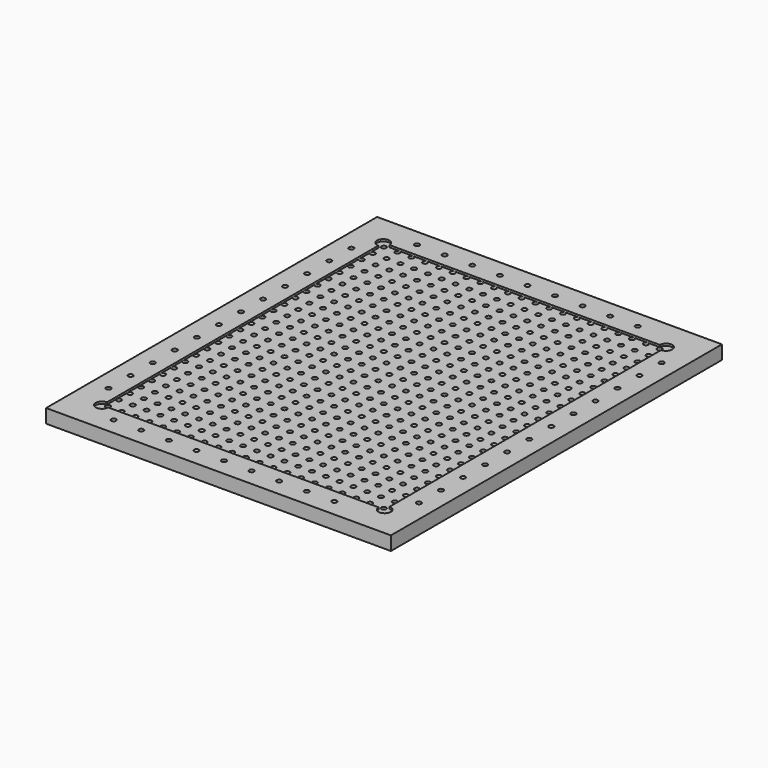
from build123d import *

# Parameters (mm, degrees)
F0_W     = 250
F0_H     = 300
F1_DEPTH = 10
F3_R     = 1.75
F4_DEPTH = 5
F5_R     = 1.75
F6_DEPTH = 5
F7_DEPTH = 1.5


with BuildPart() as f1:
    # F0 (on Top) → F1 (new body)
    with BuildSketch(Plane.XY):
        with Locations((125, 150)):
            Rectangle(F0_W, F0_H)
    extrude(amount=F1_DEPTH)

    # F3 (on face) → F4 (cut)
    with BuildSketch(Plane.XY.offset(10)):
        with Locations((24.25, 275.75)):
            Circle(F3_R)
        with Locations((24.25, 265.75)):
            Circle(F3_R)
        with Locations((24.25, 255.75)):
            Circle(F3_R)
        with Locations((24.25, 245.75)):
            Circle(F3_R)
        with Locations((24.25, 235.75)):
            Circle(F3_R)
        with Locations((24.25, 225.75)):
            Circle(F3_R)
        with Locations((24.25, 215.75)):
            Circle(F3_R)
        with Locations((24.25, 205.75)):
            Circle(F3_R)
        with Locations((24.25, 195.75)):
            Circle(F3_R)
        with Locations((24.25, 185.75)):
            Circle(F3_R)
        with Locations((24.25, 175.75)):
            Circle(F3_R)
        with Locations((24.25, 165.75)):
            Circle(F3_R)
        with Locations((24.25, 155.75)):
            Circle(F3_R)
        with Locations((24.25, 145.75)):
            Circle(F3_R)
        with Locations((24.25, 135.75)):
            Circle(F3_R)
        with Locations((24.25, 125.75)):
            Circle(F3_R)
        with Locations((24.25, 115.75)):
            Circle(F3_R)
        with Locations((24.25, 105.75)):
            Circle(F3_R)
        with Locations((24.25, 95.75)):
            Circle(F3_R)
        with Locations((24.25, 85.75)):
            Circle(F3_R)
        with Locations((24.25, 75.75)):
            Circle(F3_R)
        with Locations((24.25, 65.75)):
            Circle(F3_R)
        with Locations((24.25, 55.75)):
            Circle(F3_R)
        with Locations((24.25, 45.75)):
            Circle(F3_R)
        with Locations((24.25, 35.75)):
            Circle(F3_R)
        with Locations((24.25, 25.75)):
            Circle(F3_R)
        with Locations((34.25, 275.75)):
            Circle(F3_R)
        with Locations((34.25, 265.75)):
            Circle(F3_R)
        with Locations((34.25, 255.75)):
            Circle(F3_R)
        with Locations((34.25, 245.75)):
            Circle(F3_R)
        with Locations((34.25, 235.75)):
            Circle(F3_R)
        with Locations((34.25, 225.75)):
            Circle(F3_R)
        with Locations((34.25, 215.75)):
            Circle(F3_R)
        with Locations((34.25, 205.75)):
            Circle(F3_R)
        with Locations((34.25, 195.75)):
            Circle(F3_R)
        with Locations((34.25, 185.75)):
            Circle(F3_R)
        with Locations((34.25, 175.75)):
            Circle(F3_R)
        with Locations((34.25, 165.75)):
            Circle(F3_R)
        with Locations((34.25, 155.75)):
            Circle(F3_R)
        with Locations((34.25, 145.75)):
            Circle(F3_R)
        with Locations((34.25, 135.75)):
            Circle(F3_R)
        with Locations((34.25, 125.75)):
            Circle(F3_R)
        with Locations((34.25, 115.75)):
            Circle(F3_R)
        with Locations((34.25, 105.75)):
            Circle(F3_R)
        with Locations((34.25, 95.75)):
            Circle(F3_R)
        with Locations((34.25, 85.75)):
            Circle(F3_R)
        with Locations((34.25, 75.75)):
            Circle(F3_R)
        with Locations((34.25, 65.75)):
            Circle(F3_R)
        with Locations((34.25, 55.75)):
            Circle(F3_R)
        with Locations((34.25, 45.75)):
            Circle(F3_R)
        with Locations((34.25, 35.75)):
            Circle(F3_R)
        with Locations((34.25, 25.75)):
            Circle(F3_R)
        with Locations((44.25, 275.75)):
            Circle(F3_R)
        with Locations((44.25, 265.75)):
            Circle(F3_R)
        with Locations((44.25, 255.75)):
            Circle(F3_R)
        with Locations((44.25, 245.75)):
            Circle(F3_R)
        with Locations((44.25, 235.75)):
            Circle(F3_R)
        with Locations((44.25, 225.75)):
            Circle(F3_R)
        with Locations((44.25, 215.75)):
            Circle(F3_R)
        with Locations((44.25, 205.75)):
            Circle(F3_R)
        with Locations((44.25, 195.75)):
            Circle(F3_R)
        with Locations((44.25, 185.75)):
            Circle(F3_R)
        with Locations((44.25, 175.75)):
            Circle(F3_R)
        with Locations((44.25, 165.75)):
            Circle(F3_R)
        with Locations((44.25, 155.75)):
            Circle(F3_R)
        with Locations((44.25, 145.75)):
            Circle(F3_R)
        with Locations((44.25, 135.75)):
            Circle(F3_R)
        with Locations((44.25, 125.75)):
            Circle(F3_R)
        with Locations((44.25, 115.75)):
            Circle(F3_R)
        with Locations((44.25, 105.75)):
            Circle(F3_R)
        with Locations((44.25, 95.75)):
            Circle(F3_R)
        with Locations((44.25, 85.75)):
            Circle(F3_R)
        with Locations((44.25, 75.75)):
            Circle(F3_R)
        with Locations((44.25, 65.75)):
            Circle(F3_R)
        with Locations((44.25, 55.75)):
            Circle(F3_R)
        with Locations((44.25, 45.75)):
            Circle(F3_R)
        with Locations((44.25, 35.75)):
            Circle(F3_R)
        with Locations((44.25, 25.75)):
            Circle(F3_R)
        with Locations((54.25, 275.75)):
            Circle(F3_R)
        with Locations((54.25, 265.75)):
            Circle(F3_R)
        with Locations((54.25, 255.75)):
            Circle(F3_R)
        with Locations((54.25, 245.75)):
            Circle(F3_R)
        with Locations((54.25, 235.75)):
            Circle(F3_R)
        with Locations((54.25, 225.75)):
            Circle(F3_R)
        with Locations((54.25, 215.75)):
            Circle(F3_R)
        with Locations((54.25, 205.75)):
            Circle(F3_R)
        with Locations((54.25, 195.75)):
            Circle(F3_R)
        with Locations((54.25, 185.75)):
            Circle(F3_R)
        with Locations((54.25, 175.75)):
            Circle(F3_R)
        with Locations((54.25, 165.75)):
            Circle(F3_R)
        with Locations((54.25, 155.75)):
            Circle(F3_R)
        with Locations((54.25, 145.75)):
            Circle(F3_R)
        with Locations((54.25, 135.75)):
            Circle(F3_R)
        with Locations((54.25, 125.75)):
            Circle(F3_R)
        with Locations((54.25, 115.75)):
            Circle(F3_R)
        with Locations((54.25, 105.75)):
            Circle(F3_R)
        with Locations((54.25, 95.75)):
            Circle(F3_R)
        with Locations((54.25, 85.75)):
            Circle(F3_R)
        with Locations((54.25, 75.75)):
            Circle(F3_R)
        with Locations((54.25, 65.75)):
            Circle(F3_R)
        with Locations((54.25, 55.75)):
            Circle(F3_R)
        with Locations((54.25, 45.75)):
            Circle(F3_R)
        with Locations((54.25, 35.75)):
            Circle(F3_R)
        with Locations((54.25, 25.75)):
            Circle(F3_R)
        with Locations((64.25, 275.75)):
            Circle(F3_R)
        with Locations((64.25, 265.75)):
            Circle(F3_R)
        with Locations((64.25, 255.75)):
            Circle(F3_R)
        with Locations((64.25, 245.75)):
            Circle(F3_R)
        with Locations((64.25, 235.75)):
            Circle(F3_R)
        with Locations((64.25, 225.75)):
            Circle(F3_R)
        with Locations((64.25, 215.75)):
            Circle(F3_R)
        with Locations((64.25, 205.75)):
            Circle(F3_R)
        with Locations((64.25, 195.75)):
            Circle(F3_R)
        with Locations((64.25, 185.75)):
            Circle(F3_R)
        with Locations((64.25, 175.75)):
            Circle(F3_R)
        with Locations((64.25, 165.75)):
            Circle(F3_R)
        with Locations((64.25, 155.75)):
            Circle(F3_R)
        with Locations((64.25, 145.75)):
            Circle(F3_R)
        with Locations((64.25, 135.75)):
            Circle(F3_R)
        with Locations((64.25, 125.75)):
            Circle(F3_R)
        with Locations((64.25, 115.75)):
            Circle(F3_R)
        with Locations((64.25, 105.75)):
            Circle(F3_R)
        with Locations((64.25, 95.75)):
            Circle(F3_R)
        with Locations((64.25, 85.75)):
            Circle(F3_R)
        with Locations((64.25, 75.75)):
            Circle(F3_R)
        with Locations((64.25, 65.75)):
            Circle(F3_R)
        with Locations((64.25, 55.75)):
            Circle(F3_R)
        with Locations((64.25, 45.75)):
            Circle(F3_R)
        with Locations((64.25, 35.75)):
            Circle(F3_R)
        with Locations((64.25, 25.75)):
            Circle(F3_R)
        with Locations((74.25, 275.75)):
            Circle(F3_R)
        with Locations((74.25, 265.75)):
            Circle(F3_R)
        with Locations((74.25, 255.75)):
            Circle(F3_R)
        with Locations((74.25, 245.75)):
            Circle(F3_R)
        with Locations((74.25, 235.75)):
            Circle(F3_R)
        with Locations((74.25, 225.75)):
            Circle(F3_R)
        with Locations((74.25, 215.75)):
            Circle(F3_R)
        with Locations((74.25, 205.75)):
            Circle(F3_R)
        with Locations((74.25, 195.75)):
            Circle(F3_R)
        with Locations((74.25, 185.75)):
            Circle(F3_R)
        with Locations((74.25, 175.75)):
            Circle(F3_R)
        with Locations((74.25, 165.75)):
            Circle(F3_R)
        with Locations((74.25, 155.75)):
            Circle(F3_R)
        with Locations((74.25, 145.75)):
            Circle(F3_R)
        with Locations((74.25, 135.75)):
            Circle(F3_R)
        with Locations((74.25, 125.75)):
            Circle(F3_R)
        with Locations((74.25, 115.75)):
            Circle(F3_R)
        with Locations((74.25, 105.75)):
            Circle(F3_R)
        with Locations((74.25, 95.75)):
            Circle(F3_R)
        with Locations((74.25, 85.75)):
            Circle(F3_R)
        with Locations((74.25, 75.75)):
            Circle(F3_R)
        with Locations((74.25, 65.75)):
            Circle(F3_R)
        with Locations((74.25, 55.75)):
            Circle(F3_R)
        with Locations((74.25, 45.75)):
            Circle(F3_R)
        with Locations((74.25, 35.75)):
            Circle(F3_R)
        with Locations((74.25, 25.75)):
            Circle(F3_R)
        with Locations((84.25, 275.75)):
            Circle(F3_R)
        with Locations((84.25, 265.75)):
            Circle(F3_R)
        with Locations((84.25, 255.75)):
            Circle(F3_R)
        with Locations((84.25, 245.75)):
            Circle(F3_R)
        with Locations((84.25, 235.75)):
            Circle(F3_R)
        with Locations((84.25, 225.75)):
            Circle(F3_R)
        with Locations((84.25, 215.75)):
            Circle(F3_R)
        with Locations((84.25, 205.75)):
            Circle(F3_R)
        with Locations((84.25, 195.75)):
            Circle(F3_R)
        with Locations((84.25, 185.75)):
            Circle(F3_R)
        with Locations((84.25, 175.75)):
            Circle(F3_R)
        with Locations((84.25, 165.75)):
            Circle(F3_R)
        with Locations((84.25, 155.75)):
            Circle(F3_R)
        with Locations((84.25, 145.75)):
            Circle(F3_R)
        with Locations((84.25, 135.75)):
            Circle(F3_R)
        with Locations((84.25, 125.75)):
            Circle(F3_R)
        with Locations((84.25, 115.75)):
            Circle(F3_R)
        with Locations((84.25, 105.75)):
            Circle(F3_R)
        with Locations((84.25, 95.75)):
            Circle(F3_R)
        with Locations((84.25, 85.75)):
            Circle(F3_R)
        with Locations((84.25, 75.75)):
            Circle(F3_R)
        with Locations((84.25, 65.75)):
            Circle(F3_R)
        with Locations((84.25, 55.75)):
            Circle(F3_R)
        with Locations((84.25, 45.75)):
            Circle(F3_R)
        with Locations((84.25, 35.75)):
            Circle(F3_R)
        with Locations((84.25, 25.75)):
            Circle(F3_R)
        with Locations((94.25, 275.75)):
            Circle(F3_R)
        with Locations((94.25, 265.75)):
            Circle(F3_R)
        with Locations((94.25, 255.75)):
            Circle(F3_R)
        with Locations((94.25, 245.75)):
            Circle(F3_R)
        with Locations((94.25, 235.75)):
            Circle(F3_R)
        with Locations((94.25, 225.75)):
            Circle(F3_R)
        with Locations((94.25, 215.75)):
            Circle(F3_R)
        with Locations((94.25, 205.75)):
            Circle(F3_R)
        with Locations((94.25, 195.75)):
            Circle(F3_R)
        with Locations((94.25, 185.75)):
            Circle(F3_R)
        with Locations((94.25, 175.75)):
            Circle(F3_R)
        with Locations((94.25, 165.75)):
            Circle(F3_R)
        with Locations((94.25, 155.75)):
            Circle(F3_R)
        with Locations((94.25, 145.75)):
            Circle(F3_R)
        with Locations((94.25, 135.75)):
            Circle(F3_R)
        with Locations((94.25, 125.75)):
            Circle(F3_R)
        with Locations((94.25, 115.75)):
            Circle(F3_R)
        with Locations((94.25, 105.75)):
            Circle(F3_R)
        with Locations((94.25, 95.75)):
            Circle(F3_R)
        with Locations((94.25, 85.75)):
            Circle(F3_R)
        with Locations((94.25, 75.75)):
            Circle(F3_R)
        with Locations((94.25, 65.75)):
            Circle(F3_R)
        with Locations((94.25, 55.75)):
            Circle(F3_R)
        with Locations((94.25, 45.75)):
            Circle(F3_R)
        with Locations((94.25, 35.75)):
            Circle(F3_R)
        with Locations((94.25, 25.75)):
            Circle(F3_R)
        with Locations((104.25, 275.75)):
            Circle(F3_R)
        with Locations((104.25, 265.75)):
            Circle(F3_R)
        with Locations((104.25, 255.75)):
            Circle(F3_R)
        with Locations((104.25, 245.75)):
            Circle(F3_R)
        with Locations((104.25, 235.75)):
            Circle(F3_R)
        with Locations((104.25, 225.75)):
            Circle(F3_R)
        with Locations((104.25, 215.75)):
            Circle(F3_R)
        with Locations((104.25, 205.75)):
            Circle(F3_R)
        with Locations((104.25, 195.75)):
            Circle(F3_R)
        with Locations((104.25, 185.75)):
            Circle(F3_R)
        with Locations((104.25, 175.75)):
            Circle(F3_R)
        with Locations((104.25, 165.75)):
            Circle(F3_R)
        with Locations((104.25, 155.75)):
            Circle(F3_R)
        with Locations((104.25, 145.75)):
            Circle(F3_R)
        with Locations((104.25, 135.75)):
            Circle(F3_R)
        with Locations((104.25, 125.75)):
            Circle(F3_R)
        with Locations((104.25, 115.75)):
            Circle(F3_R)
        with Locations((104.25, 105.75)):
            Circle(F3_R)
        with Locations((104.25, 95.75)):
            Circle(F3_R)
        with Locations((104.25, 85.75)):
            Circle(F3_R)
        with Locations((104.25, 75.75)):
            Circle(F3_R)
        with Locations((104.25, 65.75)):
            Circle(F3_R)
        with Locations((104.25, 55.75)):
            Circle(F3_R)
        with Locations((104.25, 45.75)):
            Circle(F3_R)
        with Locations((104.25, 35.75)):
            Circle(F3_R)
        with Locations((104.25, 25.75)):
            Circle(F3_R)
        with Locations((114.25, 275.75)):
            Circle(F3_R)
        with Locations((114.25, 265.75)):
            Circle(F3_R)
        with Locations((114.25, 255.75)):
            Circle(F3_R)
        with Locations((114.25, 245.75)):
            Circle(F3_R)
        with Locations((114.25, 235.75)):
            Circle(F3_R)
        with Locations((114.25, 225.75)):
            Circle(F3_R)
        with Locations((114.25, 215.75)):
            Circle(F3_R)
        with Locations((114.25, 205.75)):
            Circle(F3_R)
        with Locations((114.25, 195.75)):
            Circle(F3_R)
        with Locations((114.25, 185.75)):
            Circle(F3_R)
        with Locations((114.25, 175.75)):
            Circle(F3_R)
        with Locations((114.25, 165.75)):
            Circle(F3_R)
        with Locations((114.25, 155.75)):
            Circle(F3_R)
        with Locations((114.25, 145.75)):
            Circle(F3_R)
        with Locations((114.25, 135.75)):
            Circle(F3_R)
        with Locations((114.25, 125.75)):
            Circle(F3_R)
        with Locations((114.25, 115.75)):
            Circle(F3_R)
        with Locations((114.25, 105.75)):
            Circle(F3_R)
        with Locations((114.25, 95.75)):
            Circle(F3_R)
        with Locations((114.25, 85.75)):
            Circle(F3_R)
        with Locations((114.25, 75.75)):
            Circle(F3_R)
        with Locations((114.25, 65.75)):
            Circle(F3_R)
        with Locations((114.25, 55.75)):
            Circle(F3_R)
        with Locations((114.25, 45.75)):
            Circle(F3_R)
        with Locations((114.25, 35.75)):
            Circle(F3_R)
        with Locations((114.25, 25.75)):
            Circle(F3_R)
        with Locations((124.25, 275.75)):
            Circle(F3_R)
        with Locations((124.25, 265.75)):
            Circle(F3_R)
        with Locations((124.25, 255.75)):
            Circle(F3_R)
        with Locations((124.25, 245.75)):
            Circle(F3_R)
        with Locations((124.25, 235.75)):
            Circle(F3_R)
        with Locations((124.25, 225.75)):
            Circle(F3_R)
        with Locations((124.25, 215.75)):
            Circle(F3_R)
        with Locations((124.25, 205.75)):
            Circle(F3_R)
        with Locations((124.25, 195.75)):
            Circle(F3_R)
        with Locations((124.25, 185.75)):
            Circle(F3_R)
        with Locations((124.25, 175.75)):
            Circle(F3_R)
        with Locations((124.25, 165.75)):
            Circle(F3_R)
        with Locations((124.25, 155.75)):
            Circle(F3_R)
        with Locations((124.25, 145.75)):
            Circle(F3_R)
        with Locations((124.25, 135.75)):
            Circle(F3_R)
        with Locations((124.25, 125.75)):
            Circle(F3_R)
        with Locations((124.25, 115.75)):
            Circle(F3_R)
        with Locations((124.25, 105.75)):
            Circle(F3_R)
        with Locations((124.25, 95.75)):
            Circle(F3_R)
        with Locations((124.25, 85.75)):
            Circle(F3_R)
        with Locations((124.25, 75.75)):
            Circle(F3_R)
        with Locations((124.25, 65.75)):
            Circle(F3_R)
        with Locations((124.25, 55.75)):
            Circle(F3_R)
        with Locations((124.25, 45.75)):
            Circle(F3_R)
        with Locations((124.25, 35.75)):
            Circle(F3_R)
        with Locations((124.25, 25.75)):
            Circle(F3_R)
        with Locations((134.25, 275.75)):
            Circle(F3_R)
        with Locations((134.25, 265.75)):
            Circle(F3_R)
        with Locations((134.25, 255.75)):
            Circle(F3_R)
        with Locations((134.25, 245.75)):
            Circle(F3_R)
        with Locations((134.25, 235.75)):
            Circle(F3_R)
        with Locations((134.25, 225.75)):
            Circle(F3_R)
        with Locations((134.25, 215.75)):
            Circle(F3_R)
        with Locations((134.25, 205.75)):
            Circle(F3_R)
        with Locations((134.25, 195.75)):
            Circle(F3_R)
        with Locations((134.25, 185.75)):
            Circle(F3_R)
        with Locations((134.25, 175.75)):
            Circle(F3_R)
        with Locations((134.25, 165.75)):
            Circle(F3_R)
        with Locations((134.25, 155.75)):
            Circle(F3_R)
        with Locations((134.25, 145.75)):
            Circle(F3_R)
        with Locations((134.25, 135.75)):
            Circle(F3_R)
        with Locations((134.25, 125.75)):
            Circle(F3_R)
        with Locations((134.25, 115.75)):
            Circle(F3_R)
        with Locations((134.25, 105.75)):
            Circle(F3_R)
        with Locations((134.25, 95.75)):
            Circle(F3_R)
        with Locations((134.25, 85.75)):
            Circle(F3_R)
        with Locations((134.25, 75.75)):
            Circle(F3_R)
        with Locations((134.25, 65.75)):
            Circle(F3_R)
        with Locations((134.25, 55.75)):
            Circle(F3_R)
        with Locations((134.25, 45.75)):
            Circle(F3_R)
        with Locations((134.25, 35.75)):
            Circle(F3_R)
        with Locations((134.25, 25.75)):
            Circle(F3_R)
        with Locations((144.25, 275.75)):
            Circle(F3_R)
        with Locations((144.25, 265.75)):
            Circle(F3_R)
        with Locations((144.25, 255.75)):
            Circle(F3_R)
        with Locations((144.25, 245.75)):
            Circle(F3_R)
        with Locations((144.25, 235.75)):
            Circle(F3_R)
        with Locations((144.25, 225.75)):
            Circle(F3_R)
        with Locations((144.25, 215.75)):
            Circle(F3_R)
        with Locations((144.25, 205.75)):
            Circle(F3_R)
        with Locations((144.25, 195.75)):
            Circle(F3_R)
        with Locations((144.25, 185.75)):
            Circle(F3_R)
        with Locations((144.25, 175.75)):
            Circle(F3_R)
        with Locations((144.25, 165.75)):
            Circle(F3_R)
        with Locations((144.25, 155.75)):
            Circle(F3_R)
        with Locations((144.25, 145.75)):
            Circle(F3_R)
        with Locations((144.25, 135.75)):
            Circle(F3_R)
        with Locations((144.25, 125.75)):
            Circle(F3_R)
        with Locations((144.25, 115.75)):
            Circle(F3_R)
        with Locations((144.25, 105.75)):
            Circle(F3_R)
        with Locations((144.25, 95.75)):
            Circle(F3_R)
        with Locations((144.25, 85.75)):
            Circle(F3_R)
        with Locations((144.25, 75.75)):
            Circle(F3_R)
        with Locations((144.25, 65.75)):
            Circle(F3_R)
        with Locations((144.25, 55.75)):
            Circle(F3_R)
        with Locations((144.25, 45.75)):
            Circle(F3_R)
        with Locations((144.25, 35.75)):
            Circle(F3_R)
        with Locations((144.25, 25.75)):
            Circle(F3_R)
        with Locations((154.25, 275.75)):
            Circle(F3_R)
        with Locations((154.25, 265.75)):
            Circle(F3_R)
        with Locations((154.25, 255.75)):
            Circle(F3_R)
        with Locations((154.25, 245.75)):
            Circle(F3_R)
        with Locations((154.25, 235.75)):
            Circle(F3_R)
        with Locations((154.25, 225.75)):
            Circle(F3_R)
        with Locations((154.25, 215.75)):
            Circle(F3_R)
        with Locations((154.25, 205.75)):
            Circle(F3_R)
        with Locations((154.25, 195.75)):
            Circle(F3_R)
        with Locations((154.25, 185.75)):
            Circle(F3_R)
        with Locations((154.25, 175.75)):
            Circle(F3_R)
        with Locations((154.25, 165.75)):
            Circle(F3_R)
        with Locations((154.25, 155.75)):
            Circle(F3_R)
        with Locations((154.25, 145.75)):
            Circle(F3_R)
        with Locations((154.25, 135.75)):
            Circle(F3_R)
        with Locations((154.25, 125.75)):
            Circle(F3_R)
        with Locations((154.25, 115.75)):
            Circle(F3_R)
        with Locations((154.25, 105.75)):
            Circle(F3_R)
        with Locations((154.25, 95.75)):
            Circle(F3_R)
        with Locations((154.25, 85.75)):
            Circle(F3_R)
        with Locations((154.25, 75.75)):
            Circle(F3_R)
        with Locations((154.25, 65.75)):
            Circle(F3_R)
        with Locations((154.25, 55.75)):
            Circle(F3_R)
        with Locations((154.25, 45.75)):
            Circle(F3_R)
        with Locations((154.25, 35.75)):
            Circle(F3_R)
        with Locations((154.25, 25.75)):
            Circle(F3_R)
        with Locations((164.25, 275.75)):
            Circle(F3_R)
        with Locations((164.25, 265.75)):
            Circle(F3_R)
        with Locations((164.25, 255.75)):
            Circle(F3_R)
        with Locations((164.25, 245.75)):
            Circle(F3_R)
        with Locations((164.25, 235.75)):
            Circle(F3_R)
        with Locations((164.25, 225.75)):
            Circle(F3_R)
        with Locations((164.25, 215.75)):
            Circle(F3_R)
        with Locations((164.25, 205.75)):
            Circle(F3_R)
        with Locations((164.25, 195.75)):
            Circle(F3_R)
        with Locations((164.25, 185.75)):
            Circle(F3_R)
        with Locations((164.25, 175.75)):
            Circle(F3_R)
        with Locations((164.25, 165.75)):
            Circle(F3_R)
        with Locations((164.25, 155.75)):
            Circle(F3_R)
        with Locations((164.25, 145.75)):
            Circle(F3_R)
        with Locations((164.25, 135.75)):
            Circle(F3_R)
        with Locations((164.25, 125.75)):
            Circle(F3_R)
        with Locations((164.25, 115.75)):
            Circle(F3_R)
        with Locations((164.25, 105.75)):
            Circle(F3_R)
        with Locations((164.25, 95.75)):
            Circle(F3_R)
        with Locations((164.25, 85.75)):
            Circle(F3_R)
        with Locations((164.25, 75.75)):
            Circle(F3_R)
        with Locations((164.25, 65.75)):
            Circle(F3_R)
        with Locations((164.25, 55.75)):
            Circle(F3_R)
        with Locations((164.25, 45.75)):
            Circle(F3_R)
        with Locations((164.25, 35.75)):
            Circle(F3_R)
        with Locations((164.25, 25.75)):
            Circle(F3_R)
        with Locations((174.25, 275.75)):
            Circle(F3_R)
        with Locations((174.25, 265.75)):
            Circle(F3_R)
        with Locations((174.25, 255.75)):
            Circle(F3_R)
        with Locations((174.25, 245.75)):
            Circle(F3_R)
        with Locations((174.25, 235.75)):
            Circle(F3_R)
        with Locations((174.25, 225.75)):
            Circle(F3_R)
        with Locations((174.25, 215.75)):
            Circle(F3_R)
        with Locations((174.25, 205.75)):
            Circle(F3_R)
        with Locations((174.25, 195.75)):
            Circle(F3_R)
        with Locations((174.25, 185.75)):
            Circle(F3_R)
        with Locations((174.25, 175.75)):
            Circle(F3_R)
        with Locations((174.25, 165.75)):
            Circle(F3_R)
        with Locations((174.25, 155.75)):
            Circle(F3_R)
        with Locations((174.25, 145.75)):
            Circle(F3_R)
        with Locations((174.25, 135.75)):
            Circle(F3_R)
        with Locations((174.25, 125.75)):
            Circle(F3_R)
        with Locations((174.25, 115.75)):
            Circle(F3_R)
        with Locations((174.25, 105.75)):
            Circle(F3_R)
        with Locations((174.25, 95.75)):
            Circle(F3_R)
        with Locations((174.25, 85.75)):
            Circle(F3_R)
        with Locations((174.25, 75.75)):
            Circle(F3_R)
        with Locations((174.25, 65.75)):
            Circle(F3_R)
        with Locations((174.25, 55.75)):
            Circle(F3_R)
        with Locations((174.25, 45.75)):
            Circle(F3_R)
        with Locations((174.25, 35.75)):
            Circle(F3_R)
        with Locations((174.25, 25.75)):
            Circle(F3_R)
        with Locations((184.25, 275.75)):
            Circle(F3_R)
        with Locations((184.25, 265.75)):
            Circle(F3_R)
        with Locations((184.25, 255.75)):
            Circle(F3_R)
        with Locations((184.25, 245.75)):
            Circle(F3_R)
        with Locations((184.25, 235.75)):
            Circle(F3_R)
        with Locations((184.25, 225.75)):
            Circle(F3_R)
        with Locations((184.25, 215.75)):
            Circle(F3_R)
        with Locations((184.25, 205.75)):
            Circle(F3_R)
        with Locations((184.25, 195.75)):
            Circle(F3_R)
        with Locations((184.25, 185.75)):
            Circle(F3_R)
        with Locations((184.25, 175.75)):
            Circle(F3_R)
        with Locations((184.25, 165.75)):
            Circle(F3_R)
        with Locations((184.25, 155.75)):
            Circle(F3_R)
        with Locations((184.25, 145.75)):
            Circle(F3_R)
        with Locations((184.25, 135.75)):
            Circle(F3_R)
        with Locations((184.25, 125.75)):
            Circle(F3_R)
        with Locations((184.25, 115.75)):
            Circle(F3_R)
        with Locations((184.25, 105.75)):
            Circle(F3_R)
        with Locations((184.25, 95.75)):
            Circle(F3_R)
        with Locations((184.25, 85.75)):
            Circle(F3_R)
        with Locations((184.25, 75.75)):
            Circle(F3_R)
        with Locations((184.25, 65.75)):
            Circle(F3_R)
        with Locations((184.25, 55.75)):
            Circle(F3_R)
        with Locations((184.25, 45.75)):
            Circle(F3_R)
        with Locations((184.25, 35.75)):
            Circle(F3_R)
        with Locations((184.25, 25.75)):
            Circle(F3_R)
        with Locations((194.25, 275.75)):
            Circle(F3_R)
        with Locations((194.25, 265.75)):
            Circle(F3_R)
        with Locations((194.25, 255.75)):
            Circle(F3_R)
        with Locations((194.25, 245.75)):
            Circle(F3_R)
        with Locations((194.25, 235.75)):
            Circle(F3_R)
        with Locations((194.25, 225.75)):
            Circle(F3_R)
        with Locations((194.25, 215.75)):
            Circle(F3_R)
        with Locations((194.25, 205.75)):
            Circle(F3_R)
        with Locations((194.25, 195.75)):
            Circle(F3_R)
        with Locations((194.25, 185.75)):
            Circle(F3_R)
        with Locations((194.25, 175.75)):
            Circle(F3_R)
        with Locations((194.25, 165.75)):
            Circle(F3_R)
        with Locations((194.25, 155.75)):
            Circle(F3_R)
        with Locations((194.25, 145.75)):
            Circle(F3_R)
        with Locations((194.25, 135.75)):
            Circle(F3_R)
        with Locations((194.25, 125.75)):
            Circle(F3_R)
        with Locations((194.25, 115.75)):
            Circle(F3_R)
        with Locations((194.25, 105.75)):
            Circle(F3_R)
        with Locations((194.25, 95.75)):
            Circle(F3_R)
        with Locations((194.25, 85.75)):
            Circle(F3_R)
        with Locations((194.25, 75.75)):
            Circle(F3_R)
        with Locations((194.25, 65.75)):
            Circle(F3_R)
        with Locations((194.25, 55.75)):
            Circle(F3_R)
        with Locations((194.25, 45.75)):
            Circle(F3_R)
        with Locations((194.25, 35.75)):
            Circle(F3_R)
        with Locations((194.25, 25.75)):
            Circle(F3_R)
        with Locations((204.25, 275.75)):
            Circle(F3_R)
        with Locations((204.25, 265.75)):
            Circle(F3_R)
        with Locations((204.25, 255.75)):
            Circle(F3_R)
        with Locations((204.25, 245.75)):
            Circle(F3_R)
        with Locations((204.25, 235.75)):
            Circle(F3_R)
        with Locations((204.25, 225.75)):
            Circle(F3_R)
        with Locations((204.25, 215.75)):
            Circle(F3_R)
        with Locations((204.25, 205.75)):
            Circle(F3_R)
        with Locations((204.25, 195.75)):
            Circle(F3_R)
        with Locations((204.25, 185.75)):
            Circle(F3_R)
        with Locations((204.25, 175.75)):
            Circle(F3_R)
        with Locations((204.25, 165.75)):
            Circle(F3_R)
        with Locations((204.25, 155.75)):
            Circle(F3_R)
        with Locations((204.25, 145.75)):
            Circle(F3_R)
        with Locations((204.25, 135.75)):
            Circle(F3_R)
        with Locations((204.25, 125.75)):
            Circle(F3_R)
        with Locations((204.25, 115.75)):
            Circle(F3_R)
        with Locations((204.25, 105.75)):
            Circle(F3_R)
        with Locations((204.25, 95.75)):
            Circle(F3_R)
        with Locations((204.25, 85.75)):
            Circle(F3_R)
        with Locations((204.25, 75.75)):
            Circle(F3_R)
        with Locations((204.25, 65.75)):
            Circle(F3_R)
        with Locations((204.25, 55.75)):
            Circle(F3_R)
        with Locations((204.25, 45.75)):
            Circle(F3_R)
        with Locations((204.25, 35.75)):
            Circle(F3_R)
        with Locations((204.25, 25.75)):
            Circle(F3_R)
        with Locations((214.25, 275.75)):
            Circle(F3_R)
        with Locations((214.25, 265.75)):
            Circle(F3_R)
        with Locations((214.25, 255.75)):
            Circle(F3_R)
        with Locations((214.25, 245.75)):
            Circle(F3_R)
        with Locations((214.25, 235.75)):
            Circle(F3_R)
        with Locations((214.25, 225.75)):
            Circle(F3_R)
        with Locations((214.25, 215.75)):
            Circle(F3_R)
        with Locations((214.25, 205.75)):
            Circle(F3_R)
        with Locations((214.25, 195.75)):
            Circle(F3_R)
        with Locations((214.25, 185.75)):
            Circle(F3_R)
        with Locations((214.25, 175.75)):
            Circle(F3_R)
        with Locations((214.25, 165.75)):
            Circle(F3_R)
        with Locations((214.25, 155.75)):
            Circle(F3_R)
        with Locations((214.25, 145.75)):
            Circle(F3_R)
        with Locations((214.25, 135.75)):
            Circle(F3_R)
        with Locations((214.25, 125.75)):
            Circle(F3_R)
        with Locations((214.25, 115.75)):
            Circle(F3_R)
        with Locations((214.25, 105.75)):
            Circle(F3_R)
        with Locations((214.25, 95.75)):
            Circle(F3_R)
        with Locations((214.25, 85.75)):
            Circle(F3_R)
        with Locations((214.25, 75.75)):
            Circle(F3_R)
        with Locations((214.25, 65.75)):
            Circle(F3_R)
        with Locations((214.25, 55.75)):
            Circle(F3_R)
        with Locations((214.25, 45.75)):
            Circle(F3_R)
        with Locations((214.25, 35.75)):
            Circle(F3_R)
        with Locations((214.25, 25.75)):
            Circle(F3_R)
        with Locations((224.25, 275.75)):
            Circle(F3_R)
        with Locations((224.25, 265.75)):
            Circle(F3_R)
        with Locations((224.25, 255.75)):
            Circle(F3_R)
        with Locations((224.25, 245.75)):
            Circle(F3_R)
        with Locations((224.25, 235.75)):
            Circle(F3_R)
        with Locations((224.25, 225.75)):
            Circle(F3_R)
        with Locations((224.25, 215.75)):
            Circle(F3_R)
        with Locations((224.25, 205.75)):
            Circle(F3_R)
        with Locations((224.25, 195.75)):
            Circle(F3_R)
        with Locations((224.25, 185.75)):
            Circle(F3_R)
        with Locations((224.25, 175.75)):
            Circle(F3_R)
        with Locations((224.25, 165.75)):
            Circle(F3_R)
        with Locations((224.25, 155.75)):
            Circle(F3_R)
        with Locations((224.25, 145.75)):
            Circle(F3_R)
        with Locations((224.25, 135.75)):
            Circle(F3_R)
        with Locations((224.25, 125.75)):
            Circle(F3_R)
        with Locations((224.25, 115.75)):
            Circle(F3_R)
        with Locations((224.25, 105.75)):
            Circle(F3_R)
        with Locations((224.25, 95.75)):
            Circle(F3_R)
        with Locations((224.25, 85.75)):
            Circle(F3_R)
        with Locations((224.25, 75.75)):
            Circle(F3_R)
        with Locations((224.25, 65.75)):
            Circle(F3_R)
        with Locations((224.25, 55.75)):
            Circle(F3_R)
        with Locations((224.25, 45.75)):
            Circle(F3_R)
        with Locations((224.25, 35.75)):
            Circle(F3_R)
        with Locations((224.25, 25.75)):
            Circle(F3_R)
    extrude(amount=-F4_DEPTH, mode=Mode.SUBTRACT)

    # F5 (on face) → F6 (cut)
    with BuildSketch(Plane.XY.offset(10)):
        with Locations((39, 287.5)):
            Circle(F5_R)
        with Locations((39, 12.5)):
            Circle(F5_R)
        with Locations((59, 287.5)):
            Circle(F5_R)
        with Locations((59, 12.5)):
            Circle(F5_R)
        with Locations((79, 287.5)):
            Circle(F5_R)
        with Locations((79, 12.5)):
            Circle(F5_R)
        with Locations((99, 287.5)):
            Circle(F5_R)
        with Locations((99, 12.5)):
            Circle(F5_R)
        with Locations((119, 287.5)):
            Circle(F5_R)
        with Locations((119, 12.5)):
            Circle(F5_R)
        with Locations((139, 287.5)):
            Circle(F5_R)
        with Locations((139, 12.5)):
            Circle(F5_R)
        with Locations((159, 287.5)):
            Circle(F5_R)
        with Locations((159, 12.5)):
            Circle(F5_R)
        with Locations((179, 287.5)):
            Circle(F5_R)
        with Locations((179, 12.5)):
            Circle(F5_R)
        with Locations((199, 287.5)):
            Circle(F5_R)
        with Locations((199, 12.5)):
            Circle(F5_R)
        with Locations((12.5, 261)):
            Circle(F5_R)
        with Locations((12.5, 241)):
            Circle(F5_R)
        with Locations((12.5, 221)):
            Circle(F5_R)
        with Locations((12.5, 201)):
            Circle(F5_R)
        with Locations((12.5, 181)):
            Circle(F5_R)
        with Locations((12.5, 161)):
            Circle(F5_R)
        with Locations((12.5, 141)):
            Circle(F5_R)
        with Locations((12.5, 121)):
            Circle(F5_R)
        with Locations((12.5, 101)):
            Circle(F5_R)
        with Locations((12.5, 81)):
            Circle(F5_R)
        with Locations((12.5, 61)):
            Circle(F5_R)
        with Locations((12.5, 41)):
            Circle(F5_R)
        with Locations((237.5, 261)):
            Circle(F5_R)
        with Locations((237.5, 241)):
            Circle(F5_R)
        with Locations((237.5, 221)):
            Circle(F5_R)
        with Locations((237.5, 201)):
            Circle(F5_R)
        with Locations((237.5, 181)):
            Circle(F5_R)
        with Locations((237.5, 161)):
            Circle(F5_R)
        with Locations((237.5, 141)):
            Circle(F5_R)
        with Locations((237.5, 121)):
            Circle(F5_R)
        with Locations((237.5, 101)):
            Circle(F5_R)
        with Locations((237.5, 81)):
            Circle(F5_R)
        with Locations((237.5, 61)):
            Circle(F5_R)
        with Locations((237.5, 41)):
            Circle(F5_R)
    extrude(amount=-F6_DEPTH, mode=Mode.SUBTRACT)

    # F2 (on face) → F7 (cut)
    with BuildSketch(Plane.XY.offset(10)):
        with BuildLine():
            Line((22.5, 273), (22.5, 277.5))
            Line((22.5, 277.5), (27, 277.5))
            ThreePointArc((27, 277.5), (19.3180194847, 280.6819805153), (22.5, 273))
        make_face()
        with BuildLine():
            Line((27, 277.5), (22.5, 277.5))
            Line((22.5, 277.5), (22.5, 273))
            ThreePointArc((22.5, 273), (25.6819805153, 274.3180194847), (27, 277.5))
        make_face()
        with BuildLine():
            Line((223, 277.5), (27, 277.5))
            ThreePointArc((27, 277.5), (25.6819805153, 274.3180194847), (22.5, 273))
            Line((22.5, 273), (22.5, 27))
            ThreePointArc((22.5, 27), (25.6819805153, 25.6819805153), (27, 22.5))
            Line((27, 22.5), (223, 22.5))
            ThreePointArc((223, 22.5), (224.3180194847, 25.6819805153), (227.5, 27))
            Line((227.5, 27), (227.5, 273))
            ThreePointArc((227.5, 273), (224.3180194847, 274.3180194847), (223, 277.5))
        make_face()
        with BuildLine():
            ThreePointArc((232, 277.5), (227.5, 282), (223, 277.5))
            Line((223, 277.5), (227.5, 277.5))
            Line((227.5, 277.5), (227.5, 273))
            ThreePointArc((227.5, 273), (230.6819805153, 274.3180194847), (232, 277.5))
        make_face()
        with BuildLine():
            Line((227.5, 277.5), (223, 277.5))
            ThreePointArc((223, 277.5), (224.3180194847, 274.3180194847), (227.5, 273))
            Line((227.5, 273), (227.5, 277.5))
        make_face()
        with BuildLine():
            ThreePointArc((27, 22.5), (25.6819805153, 25.6819805153), (22.5, 27))
            Line((22.5, 27), (22.5, 22.5))
            Line((22.5, 22.5), (27, 22.5))
        make_face()
        with BuildLine():
            Line((22.5, 22.5), (22.5, 27))
            ThreePointArc((22.5, 27), (19.3180194847, 19.3180194847), (27, 22.5))
            Line((27, 22.5), (22.5, 22.5))
        make_face()
        with BuildLine():
            ThreePointArc((232, 22.5), (230.6819805153, 25.6819805153), (227.5, 27))
            Line((227.5, 27), (227.5, 22.5))
            Line((227.5, 22.5), (223, 22.5))
            ThreePointArc((223, 22.5), (227.5, 18), (232, 22.5))
        make_face()
        with BuildLine():
            Line((227.5, 22.5), (227.5, 27))
            ThreePointArc((227.5, 27), (224.3180194847, 25.6819805153), (223, 22.5))
            Line((223, 22.5), (227.5, 22.5))
        make_face()
    extrude(amount=-F7_DEPTH, mode=Mode.SUBTRACT)


solid = f1.part
